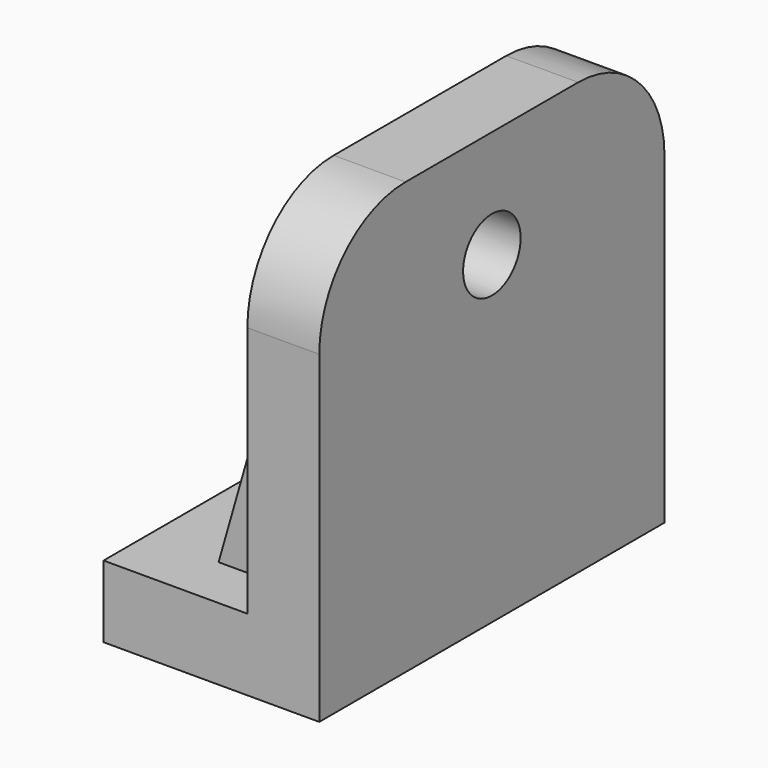
from build123d import *

# Parameters (mm, degrees)
F1_DEPTH  = 76.2
F2_R      = 12.7
F3_DEPTH  = 76.201
F5_DEPTH  = 46.736
F6_R      = 19.05
F7_DEPTH  = 6.35
F8_R      = 38.1
F11_DEPTH = 12.7


# Not quite as in the source:
# - a pattern or mirror of a feature is missing from the dataset's text; its kind, count and spacing are read off the source's solid


with BuildPart() as f1:
    # F0 (on Front) → F1 (new body, symmetric)
    with BuildSketch(Plane.XZ):
        Polygon((-76.2, 0), (0, 0), (0, 152.4), (-25.4, 152.4), (-25.4, 25.4), (-76.2, 25.4), align=None)
    extrude(amount=F1_DEPTH, both=True)

    # F2 (on Right) → F3 (cut, through all)
    with BuildSketch(Plane.YZ):
        with Locations((0, 114.3)):
            Circle(F2_R)
    extrude(amount=-F3_DEPTH, mode=Mode.SUBTRACT)

    # F4 (on face) → F5 (cut)
    with BuildSketch(Plane.XY.offset(25.4)):
        with BuildLine():
            ThreePointArc((-63.5, -12.7), (-54.5197438789, -8.9802561211), (-50.8, 0))
            ThreePointArc((-50.8, 0), (-54.5197438789, 8.9802561211), (-63.5, 12.7))
            Line((-63.5, 12.7), (-76.2, 12.7))
            Line((-76.2, 12.7), (-76.2, -12.7))
            Line((-76.2, -12.7), (-63.5, -12.7))
        make_face()
    extrude(amount=-F5_DEPTH, mode=Mode.SUBTRACT)

    # F6 (on face) → F7 (cut)
    with BuildSketch(Plane(origin=(-25.4, 0, 0), x_dir=(0, -1, 0), z_dir=(-1, 0, 0))):
        with Locations((-0.0589386239, 113.8949071477)):
            Circle(F6_R)
    extrude(amount=-F7_DEPTH, mode=Mode.SUBTRACT)

    # F8
    f8_edges = [f1.edges().sort_by_distance(p)[0] for p in [
        (-12.7, 76.2, 152.4),
        (-12.7, -76.2, 152.4),
    ]]
    fillet(f8_edges, radius=F8_R)

    # F10 (on offset) → F11 (join)
    with BuildSketch(Plane.XZ.offset(44.45)):
        Polygon((-25.4, 25.4), (-25.4, 114.3), (-50.8, 25.4), align=None)
    f11 = extrude(amount=F11_DEPTH)

    # F11_copies: F11 across plane
    add(f11.mirror(Plane.ZX))


solid = f1.part
